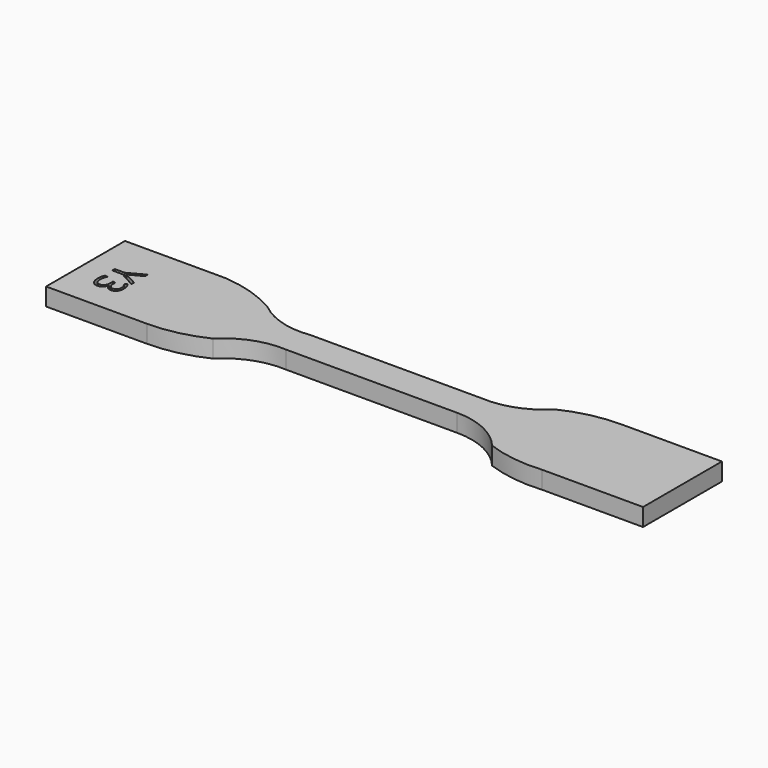
from build123d import *

# Parameters (mm, degrees)
F1_DEPTH     = 3.4
F2_TEXT_SIZE = 7.0564552314
F3_DEPTH     = 1


# Not quite as in the source:
# - Text() gives the source's letters only with a copy of the font that has no kerning and outlines rounded to 1/6400 em; it was checked with that copy


with BuildPart() as f1:
    # F0 (on Top) → F1 (new body)
    with BuildSketch(Plane.XY):
        with BuildLine():
            Line((-14.4320548165, 19.7811394548), (-33.8720548165, 19.7811394548))
            Line((-33.8720548165, 19.7811394548), (-33.8720548165, 0.7811394548))
            Line((-33.8720548165, 0.7811394548), (-14.4320548165, 0.7811394548))
            ThreePointArc((-14.4320548165, 0.7811394548), (-8.9053122052, 1.3996892086), (-3.6520548165, 3.2247301661))
            ThreePointArc((-3.6520548165, 3.2247301661), (1.3014698263, 6.4128780055), (7.1279451835, 7.2811394548))
            Line((7.1279451835, 7.2811394548), (40.1279451835, 7.2811394548))
            ThreePointArc((40.1279451835, 7.2811394548), (46.0837574042, 5.9511158081), (50.9079451835, 2.2137538538))
            ThreePointArc((50.9079451835, 2.2137538538), (56.2191047011, 0.9041953221), (61.6879451835, 0.7811394548))
            Line((61.6879451835, 0.7811394548), (81.1279451835, 0.7811394548))
            Line((81.1279451835, 0.7811394548), (81.1279451835, 19.7811394548))
            Line((81.1279451835, 19.7811394548), (61.6879451835, 19.7811394548))
            ThreePointArc((61.6879451835, 19.7811394548), (56.1612025723, 19.162589701), (50.9079451835, 17.3375487435))
            ThreePointArc((50.9079451835, 17.3375487435), (45.9544205407, 14.1494009041), (40.1279451835, 13.2811394548))
            Line((40.1279451835, 13.2811394548), (7.1279451835, 13.2811394548))
            ThreePointArc((7.1279451835, 13.2811394548), (1.4167452884, 13.6925537245), (-3.6520548165, 16.3560723447))
            ThreePointArc((-3.6520548165, 16.3560723447), (-8.8458057958, 18.686276846), (-14.4320548165, 19.7811394548))
        make_face()
    extrude(amount=F1_DEPTH)

    # F2 (on face) → F3 (cut)
    with BuildSketch(Plane.XY.offset(3.4)):
        with Locations(Location((-29.3720550835, 13.353464842), (0, 0, -90))):
            Text('Y3', F2_TEXT_SIZE, font='Open Sans', text_align=(TextAlign.LEFT, TextAlign.BOTTOM))
    extrude(amount=-F3_DEPTH, mode=Mode.SUBTRACT)


solid = f1.part
